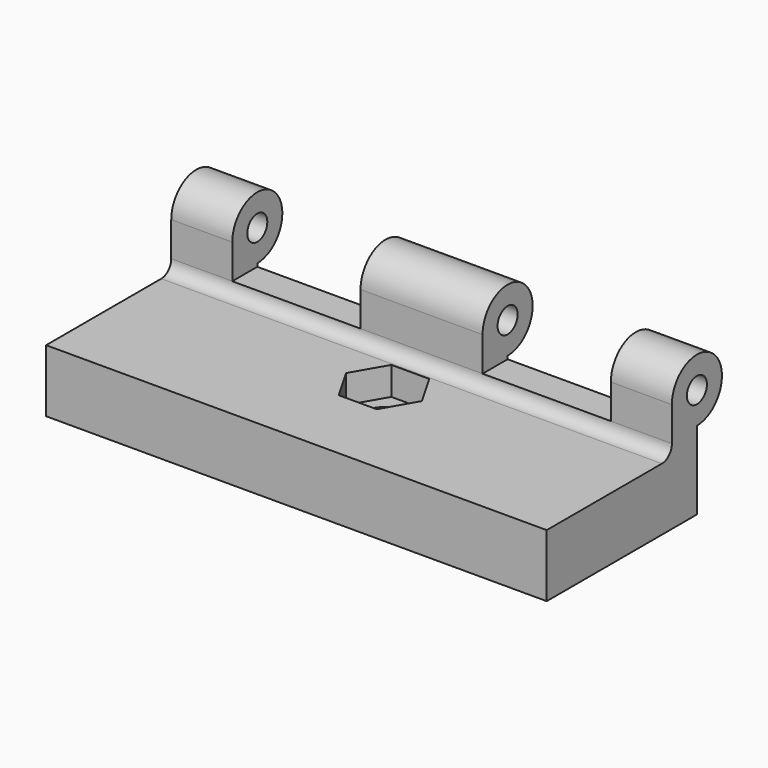
from build123d import *

# Parameters (mm, degrees)
F1_DEPTH  = 40
F2_R      = 2
F3_DEPTH  = 80.001
F4_R      = 2
F6_W      = 20.5
F6_H      = 12
F7_DEPTH  = 10.501
F9_DEPTH  = 4.5
F10_R     = 3.25
F11_DEPTH = 22.501


# Not quite as in the source:
# - a pattern or mirror of a feature is missing from the dataset's text; its kind, count and spacing are read off the source's solid


with BuildPart() as f1:
    # F0 (on Right) → F1 (new body, symmetric)
    with BuildSketch(Plane.YZ):
        with BuildLine():
            Line((-17.5, 10), (-17.5, 0))
            Line((-17.5, 0), (12.5, 0))
            Line((12.5, 0), (12.5, 12.5))
            ThreePointArc((12.5, 12.5), (16.0355339059, 21.0355339059), (7.5, 17.5))
            Line((7.5, 17.5), (7.5, 10))
            Line((7.5, 10), (-17.5, 10))
        make_face()
    extrude(amount=F1_DEPTH, both=True)

    # F2 (on face) → F3 (cut, through all)
    with BuildSketch(Plane.YZ.offset(40)):
        with Locations((12.5, 17.5)):
            Circle(F2_R)
    extrude(amount=-F3_DEPTH, mode=Mode.SUBTRACT)

    # F4
    f4_edges = [f1.edges().sort_by_distance(p)[0] for p in [
        (0, 7.5, 10),
    ]]
    fillet(f4_edges, radius=F4_R)

    # F6 (on offset) → F7 (cut, through all)
    with BuildSketch(Plane.XY.offset(12)):
        with Locations((20, 13.5)):
            Rectangle(F6_W, F6_H)
    f7 = extrude(amount=F7_DEPTH, mode=Mode.SUBTRACT)

    # F7_copies: F7 across plane
    add(f7.mirror(Plane(origin=(0, 0, 0), x_dir=(0, 0, -1), z_dir=(-1, 0, 0))), mode=Mode.SUBTRACT)

    # F8 (on face) → F9 (cut)
    with BuildSketch(Plane.XY.offset(10)):
        Polygon((-3.0310889132, -5.25), (3.0310889132, -5.25), (6.0621778265, 0), (3.0310889132, 5.25), (-3.0310889132, 5.25), (-6.0621778265, 0), align=None)
    extrude(amount=-F9_DEPTH, mode=Mode.SUBTRACT)

    # F10 (on face) → F11 (cut, through all)
    with BuildSketch(Plane(origin=(0, 0, 0), x_dir=(1, 0, 0), z_dir=(0, 0, -1))):
        Circle(F10_R)
    extrude(amount=-F11_DEPTH, mode=Mode.SUBTRACT)


solid = f1.part
